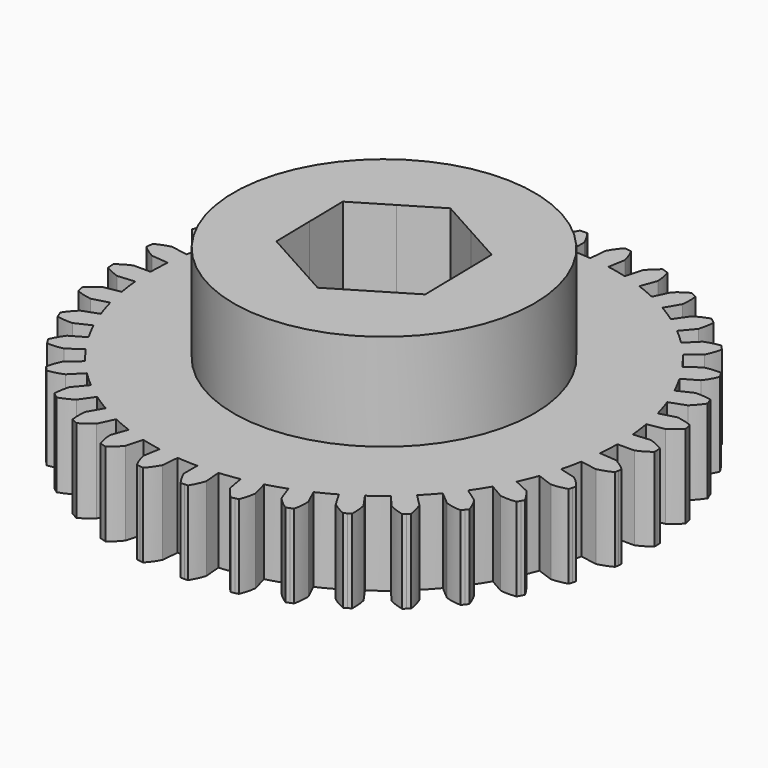
from build123d import *

# Parameters (mm, degrees)
F1_DEPTH = 6.35
F2_R     = 11.43
F3_DEPTH = 7.366
F5_DEPTH = 25.4


with BuildPart() as f1:
    # F0 (on Top) → F1 (new body)
    with BuildSketch(Plane.XY):
        with BuildLine():
            ThreePointArc((0, 19.05), (-0.2695882534, 19.591766176), (-0.6056993608, 20.0949736276))
            ThreePointArc((-0.6056993608, 20.0949736276), (-0.7413308329, 20.0904272082), (-0.8769285255, 20.0849653515))
            ThreePointArc((-0.8769285255, 20.0849653515), (-1.0124862602, 20.0785883065), (-1.1479978601, 20.0712963638))
            ThreePointArc((-1.1479978601, 20.0712963638), (-1.4389725441, 19.5407097553), (-1.6603168993, 18.9775089986))
            Line((-1.6603168993, 18.9775089986), (-1.5474284157, 17.6871877261))
            ThreePointArc((-1.5474284157, 17.6871877261), (-2.3174598996, 17.6028555631), (-3.0830799668, 17.485015364))
            Line((-3.0830799668, 17.485015364), (-3.3079977846, 18.7605876949))
            ThreePointArc((-3.3079977846, 18.7605876949), (-3.6675670958, 19.2473097165), (-4.0859529772, 19.6845072348))
            ThreePointArc((-4.0859529772, 19.6845072348), (-4.218734425, 19.6564777277), (-4.3513236426, 19.6275525567))
            ThreePointArc((-4.3513236426, 19.6275525567), (-4.4837145884, 19.5977330398), (-4.6159012301, 19.5670205357))
            ThreePointArc((-4.6159012301, 19.5670205357), (-4.8103199572, 18.9939675064), (-4.9305028092, 18.4008869908))
            Line((-4.9305028092, 18.4008869908), (-4.5952674177, 17.1497714772))
            ThreePointArc((-4.5952674177, 17.1497714772), (-5.3389562666, 16.9330059453), (-6.0724821089, 16.6840074742))
            Line((-6.0724821089, 16.6840074742), (-6.5154837304, 17.901144426))
            ThreePointArc((-6.5154837304, 17.901144426), (-6.9541087679, 18.3180334907), (-7.44205698, 18.6759370506))
            ThreePointArc((-7.44205698, 18.6759370506), (-7.5679539064, 18.6252761182), (-7.6935059926, 18.5737665096))
            ThreePointArc((-7.6935059926, 18.5737665096), (-7.8187075178, 18.5214105716), (-7.9435527769, 18.46821069))
            ThreePointArc((-7.9435527769, 18.46821069), (-8.0355082324, 17.8701031662), (-8.0508778862, 17.265163343))
            Line((-8.0508778862, 17.265163343), (-7.5034815445, 16.0912681002))
            ThreePointArc((-7.5034815445, 16.0912681002), (-8.1982311492, 15.7486555104), (-8.8773749549, 15.3760644598))
            Line((-8.8773749549, 15.3760644598), (-9.525, 16.4977839421))
            ThreePointArc((-9.525, 16.4977839421), (-10.029353364, 16.8321730868), (-10.5720378473, 17.0999079695))
            ThreePointArc((-10.5720378473, 17.0999079695), (-10.6872249379, 17.0281549187), (-10.8019250562, 16.9556259658))
            ThreePointArc((-10.8019250562, 16.9556259658), (-10.9161329756, 16.8823244155), (-11.0298434923, 16.8082536079))
            ThreePointArc((-11.0298434923, 16.8082536079), (-11.0165416562, 16.203264784), (-10.9266311125, 15.6048464437))
            Line((-10.9266311125, 15.6048464437), (-10.1837061816, 14.5438396845))
            ThreePointArc((-10.1837061816, 14.5438396845), (-10.8084069268, 14.085790147), (-11.4125332551, 13.6009275074))
            Line((-11.4125332551, 13.6009275074), (-12.2451039645, 14.5931466414))
            ThreePointArc((-12.2451039645, 14.5931466414), (-12.7998611333, 14.8348756211), (-13.3807926944, 15.0043068377))
            ThreePointArc((-13.3807926944, 15.0043068377), (-13.4817700477, 14.9136418487), (-13.5821330929, 14.822297307))
            ThreePointArc((-13.5821330929, 14.822297307), (-13.6818772568, 14.7302773748), (-13.7809979945, 14.6375862452))
            ThreePointArc((-13.7809979945, 14.6375862452), (-13.6628430364, 14.0440984006), (-13.4703841816, 13.4703841816))
            Line((-13.4703841816, 13.4703841816), (-12.5545040595, 12.5545040595))
            ThreePointArc((-12.5545040595, 12.5545040595), (-13.0901747293, 11.9949351778), (-13.6009275074, 11.4125332551))
            Line((-13.6009275074, 11.4125332551), (-14.5931466414, 12.2451039645))
            ThreePointArc((-14.5931466414, 12.2451039645), (-15.181451599, 12.3868279664), (-15.7829789264, 12.4528074353))
            ThreePointArc((-15.7829789264, 12.4528074353), (-15.8666783967, 12.3459853177), (-15.9496548885, 12.2386006449))
            ThreePointArc((-15.9496548885, 12.2386006449), (-16.0319046209, 12.1306583101), (-16.1134238461, 12.0221632315))
            ThreePointArc((-16.1134238461, 12.0221632315), (-15.8940058447, 11.4582091939), (-15.6048464437, 10.9266311125))
            Line((-15.6048464437, 10.9266311125), (-14.5438396845, 10.1837061816))
            ThreePointArc((-14.5438396845, 10.1837061816), (-14.9742041965, 9.5396201729), (-15.3760644598, 8.8773749549))
            Line((-15.3760644598, 8.8773749549), (-16.4977839421, 9.525))
            ThreePointArc((-16.4977839421, 9.525), (-17.1017613401, 9.562412812), (-17.7056073303, 9.5229357803))
            ThreePointArc((-17.7056073303, 9.5229357803), (-17.7694857516, 9.4032022702), (-17.8325544913, 9.2830402953))
            ThreePointArc((-17.8325544913, 9.2830402953), (-17.8948106757, 9.1624553309), (-17.956251468, 9.0414528715))
            ThreePointArc((-17.956251468, 9.0414528715), (-17.6422373281, 8.5241680991), (-17.265163343, 8.0508778862))
            Line((-17.265163343, 8.0508778862), (-16.0912681002, 7.5034815445))
            ThreePointArc((-16.0912681002, 7.5034815445), (-16.4032500466, 6.7944486363), (-16.6840074742, 6.0724821089))
            Line((-16.6840074742, 6.0724821089), (-17.901144426, 6.5154837304))
            ThreePointArc((-17.901144426, 6.5154837304), (-18.5024427168, 6.4474485832), (-19.0902598149, 6.3037145405))
            ThreePointArc((-19.0902598149, 6.3037145405), (-19.1323762736, 6.17470768), (-19.1736209495, 6.0454194638))
            ThreePointArc((-19.1736209495, 6.0454194638), (-19.2139919633, 5.915855783), (-19.2534874753, 5.7860225412))
            ThreePointArc((-19.2534874753, 5.7860225412), (-18.8544183577, 5.33112447), (-18.4008869908, 4.9305028092))
            Line((-18.4008869908, 4.9305028092), (-17.1497714772, 4.5952674177))
            ThreePointArc((-17.1497714772, 4.5952674177), (-17.3338914444, 3.8428312161), (-17.485015364, 3.0830799668))
            Line((-17.485015364, 3.0830799668), (-18.7605876949, 3.3079977846))
            ThreePointArc((-18.7605876949, 3.3079977846), (-19.3409367343, 3.1365818917), (-19.8948644153, 2.8929581242))
            ThreePointArc((-19.8948644153, 2.8929581242), (-19.9139392241, 2.7585977215), (-19.9321066375, 2.624111621))
            ThreePointArc((-19.9321066375, 2.624111621), (-19.9493658278, 2.4895059507), (-19.9657160084, 2.3547868439))
            ThreePointArc((-19.9657160084, 2.3547868439), (-19.4937174264, 1.9760973215), (-18.9775089986, 1.6603168993))
            Line((-18.9775089986, 1.6603168993), (-17.6871877261, 1.5474284157))
            ThreePointArc((-17.6871877261, 1.5474284157), (-17.7378513221, 0.7744513139), (-17.7547499098, 0))
            Line((-17.7547499098, 0), (-19.05, 0))
            ThreePointArc((-19.05, 0), (-19.591766176, -0.2695882534), (-20.0949736276, -0.6056993608))
            ThreePointArc((-20.0949736276, -0.6056993608), (-20.0904272082, -0.7413308329), (-20.0849653515, -0.8769285255))
            ThreePointArc((-20.0849653515, -0.8769285255), (-20.0785883065, -1.0124862602), (-20.0712963638, -1.1479978601))
            ThreePointArc((-20.0712963638, -1.1479978601), (-19.5407097553, -1.4389725441), (-18.9775089986, -1.6603168993))
            Line((-18.9775089986, -1.6603168993), (-17.6871877261, -1.5474284157))
            ThreePointArc((-17.6871877261, -1.5474284157), (-17.6028555631, -2.3174598996), (-17.485015364, -3.0830799668))
            Line((-17.485015364, -3.0830799668), (-18.7605876949, -3.3079977846))
            ThreePointArc((-18.7605876949, -3.3079977846), (-19.2473097165, -3.6675670958), (-19.6845072348, -4.0859529772))
            ThreePointArc((-19.6845072348, -4.0859529772), (-19.6564777277, -4.218734425), (-19.6275525567, -4.3513236426))
            ThreePointArc((-19.6275525567, -4.3513236426), (-19.5977330398, -4.4837145884), (-19.5670205357, -4.6159012301))
            ThreePointArc((-19.5670205357, -4.6159012301), (-18.9939675064, -4.8103199572), (-18.4008869908, -4.9305028092))
            Line((-18.4008869908, -4.9305028092), (-17.1497714772, -4.5952674177))
            ThreePointArc((-17.1497714772, -4.5952674177), (-16.9330059453, -5.3389562666), (-16.6840074742, -6.0724821089))
            Line((-16.6840074742, -6.0724821089), (-17.901144426, -6.5154837304))
            ThreePointArc((-17.901144426, -6.5154837304), (-18.3180334907, -6.9541087679), (-18.6759370506, -7.44205698))
            ThreePointArc((-18.6759370506, -7.44205698), (-18.6252761182, -7.5679539064), (-18.5737665096, -7.6935059926))
            ThreePointArc((-18.5737665096, -7.6935059926), (-18.5214105716, -7.8187075178), (-18.46821069, -7.9435527769))
            ThreePointArc((-18.46821069, -7.9435527769), (-17.8701031662, -8.0355082324), (-17.265163343, -8.0508778862))
            Line((-17.265163343, -8.0508778862), (-16.0912681002, -7.5034815445))
            ThreePointArc((-16.0912681002, -7.5034815445), (-15.7486555104, -8.1982311492), (-15.3760644598, -8.8773749549))
            Line((-15.3760644598, -8.8773749549), (-16.4977839421, -9.525))
            ThreePointArc((-16.4977839421, -9.525), (-16.8321730868, -10.029353364), (-17.0999079695, -10.5720378473))
            ThreePointArc((-17.0999079695, -10.5720378473), (-17.0281549187, -10.6872249379), (-16.9556259658, -10.8019250562))
            ThreePointArc((-16.9556259658, -10.8019250562), (-16.8823244155, -10.9161329756), (-16.8082536079, -11.0298434923))
            ThreePointArc((-16.8082536079, -11.0298434923), (-16.203264784, -11.0165416562), (-15.6048464437, -10.9266311125))
            Line((-15.6048464437, -10.9266311125), (-14.5438396845, -10.1837061816))
            ThreePointArc((-14.5438396845, -10.1837061816), (-14.085790147, -10.8084069268), (-13.6009275074, -11.4125332551))
            Line((-13.6009275074, -11.4125332551), (-14.5931466414, -12.2451039645))
            ThreePointArc((-14.5931466414, -12.2451039645), (-14.8348756211, -12.7998611333), (-15.0043068377, -13.3807926944))
            ThreePointArc((-15.0043068377, -13.3807926944), (-14.9136418487, -13.4817700477), (-14.822297307, -13.5821330929))
            ThreePointArc((-14.822297307, -13.5821330929), (-14.7302773748, -13.6818772568), (-14.6375862452, -13.7809979945))
            ThreePointArc((-14.6375862452, -13.7809979945), (-14.0440984006, -13.6628430364), (-13.4703841816, -13.4703841816))
            Line((-13.4703841816, -13.4703841816), (-12.5545040595, -12.5545040595))
            ThreePointArc((-12.5545040595, -12.5545040595), (-11.9949351778, -13.0901747293), (-11.4125332551, -13.6009275074))
            Line((-11.4125332551, -13.6009275074), (-12.2451039645, -14.5931466414))
            ThreePointArc((-12.2451039645, -14.5931466414), (-12.3868279664, -15.181451599), (-12.4528074353, -15.7829789264))
            ThreePointArc((-12.4528074353, -15.7829789264), (-12.3459853177, -15.8666783967), (-12.2386006449, -15.9496548885))
            ThreePointArc((-12.2386006449, -15.9496548885), (-12.1306583101, -16.0319046209), (-12.0221632315, -16.1134238461))
            ThreePointArc((-12.0221632315, -16.1134238461), (-11.4582091939, -15.8940058447), (-10.9266311125, -15.6048464437))
            Line((-10.9266311125, -15.6048464437), (-10.1837061816, -14.5438396845))
            ThreePointArc((-10.1837061816, -14.5438396845), (-9.5396201729, -14.9742041965), (-8.8773749549, -15.3760644598))
            Line((-8.8773749549, -15.3760644598), (-9.525, -16.4977839421))
            ThreePointArc((-9.525, -16.4977839421), (-9.562412812, -17.1017613401), (-9.5229357803, -17.7056073303))
            ThreePointArc((-9.5229357803, -17.7056073303), (-9.4032022702, -17.7694857516), (-9.2830402953, -17.8325544913))
            ThreePointArc((-9.2830402953, -17.8325544913), (-9.1624553309, -17.8948106757), (-9.0414528715, -17.956251468))
            ThreePointArc((-9.0414528715, -17.956251468), (-8.5241680991, -17.6422373281), (-8.0508778862, -17.265163343))
            Line((-8.0508778862, -17.265163343), (-7.5034815445, -16.0912681002))
            ThreePointArc((-7.5034815445, -16.0912681002), (-6.7944486363, -16.4032500466), (-6.0724821089, -16.6840074742))
            Line((-6.0724821089, -16.6840074742), (-6.5154837304, -17.901144426))
            ThreePointArc((-6.5154837304, -17.901144426), (-6.4474485832, -18.5024427168), (-6.3037145405, -19.0902598149))
            ThreePointArc((-6.3037145405, -19.0902598149), (-6.17470768, -19.1323762736), (-6.0454194638, -19.1736209495))
            ThreePointArc((-6.0454194638, -19.1736209495), (-5.915855783, -19.2139919633), (-5.7860225412, -19.2534874753))
            ThreePointArc((-5.7860225412, -19.2534874753), (-5.33112447, -18.8544183577), (-4.9305028092, -18.4008869908))
            Line((-4.9305028092, -18.4008869908), (-4.5952674177, -17.1497714772))
            ThreePointArc((-4.5952674177, -17.1497714772), (-3.8428312161, -17.3338914444), (-3.0830799668, -17.485015364))
            Line((-3.0830799668, -17.485015364), (-3.3079977846, -18.7605876949))
            ThreePointArc((-3.3079977846, -18.7605876949), (-3.1365818917, -19.3409367343), (-2.8929581242, -19.8948644153))
            ThreePointArc((-2.8929581242, -19.8948644153), (-2.7585977215, -19.9139392241), (-2.624111621, -19.9321066375))
            ThreePointArc((-2.624111621, -19.9321066375), (-2.4895059507, -19.9493658278), (-2.3547868439, -19.9657160084))
            ThreePointArc((-2.3547868439, -19.9657160084), (-1.9760973215, -19.4937174264), (-1.6603168993, -18.9775089986))
            Line((-1.6603168993, -18.9775089986), (-1.5474284157, -17.6871877261))
            ThreePointArc((-1.5474284157, -17.6871877261), (-0.7744513139, -17.7378513221), (0, -17.7547499098))
            Line((0, -17.7547499098), (0, -19.05))
            ThreePointArc((0, -19.05), (0.2695882534, -19.591766176), (0.6056993608, -20.0949736276))
            ThreePointArc((0.6056993608, -20.0949736276), (0.7413308329, -20.0904272082), (0.8769285255, -20.0849653515))
            ThreePointArc((0.8769285255, -20.0849653515), (1.0124862602, -20.0785883065), (1.1479978601, -20.0712963638))
            ThreePointArc((1.1479978601, -20.0712963638), (1.4389725441, -19.5407097553), (1.6603168993, -18.9775089986))
            Line((1.6603168993, -18.9775089986), (1.5474284157, -17.6871877261))
            ThreePointArc((1.5474284157, -17.6871877261), (2.3174598996, -17.6028555631), (3.0830799668, -17.485015364))
            Line((3.0830799668, -17.485015364), (3.3079977846, -18.7605876949))
            ThreePointArc((3.3079977846, -18.7605876949), (3.6675670958, -19.2473097165), (4.0859529772, -19.6845072348))
            ThreePointArc((4.0859529772, -19.6845072348), (4.218734425, -19.6564777277), (4.3513236426, -19.6275525567))
            ThreePointArc((4.3513236426, -19.6275525567), (4.4837145884, -19.5977330398), (4.6159012301, -19.5670205357))
            ThreePointArc((4.6159012301, -19.5670205357), (4.8103199572, -18.9939675064), (4.9305028092, -18.4008869908))
            Line((4.9305028092, -18.4008869908), (4.5952674177, -17.1497714772))
            ThreePointArc((4.5952674177, -17.1497714772), (5.3389562666, -16.9330059453), (6.0724821089, -16.6840074742))
            Line((6.0724821089, -16.6840074742), (6.5154837304, -17.901144426))
            ThreePointArc((6.5154837304, -17.901144426), (6.9541087679, -18.3180334907), (7.44205698, -18.6759370506))
            ThreePointArc((7.44205698, -18.6759370506), (7.5679539064, -18.6252761182), (7.6935059926, -18.5737665096))
            ThreePointArc((7.6935059926, -18.5737665096), (7.8187075178, -18.5214105716), (7.9435527769, -18.46821069))
            ThreePointArc((7.9435527769, -18.46821069), (8.0355082324, -17.8701031662), (8.0508778862, -17.265163343))
            Line((8.0508778862, -17.265163343), (7.5034815445, -16.0912681002))
            ThreePointArc((7.5034815445, -16.0912681002), (8.1982311492, -15.7486555104), (8.8773749549, -15.3760644598))
            Line((8.8773749549, -15.3760644598), (9.525, -16.4977839421))
            ThreePointArc((9.525, -16.4977839421), (10.029353364, -16.8321730868), (10.5720378473, -17.0999079695))
            ThreePointArc((10.5720378473, -17.0999079695), (10.6872249379, -17.0281549187), (10.8019250562, -16.9556259658))
            ThreePointArc((10.8019250562, -16.9556259658), (10.9161329756, -16.8823244155), (11.0298434923, -16.8082536079))
            ThreePointArc((11.0298434923, -16.8082536079), (11.0165416562, -16.203264784), (10.9266311125, -15.6048464437))
            Line((10.9266311125, -15.6048464437), (10.1837061816, -14.5438396845))
            ThreePointArc((10.1837061816, -14.5438396845), (10.8084069268, -14.085790147), (11.4125332551, -13.6009275074))
            Line((11.4125332551, -13.6009275074), (12.2451039645, -14.5931466414))
            ThreePointArc((12.2451039645, -14.5931466414), (12.7998611333, -14.8348756211), (13.3807926944, -15.0043068377))
            ThreePointArc((13.3807926944, -15.0043068377), (13.4817700477, -14.9136418487), (13.5821330929, -14.822297307))
            ThreePointArc((13.5821330929, -14.822297307), (13.6818772568, -14.7302773748), (13.7809979945, -14.6375862452))
            ThreePointArc((13.7809979945, -14.6375862452), (13.6628430364, -14.0440984006), (13.4703841816, -13.4703841816))
            Line((13.4703841816, -13.4703841816), (12.5545040595, -12.5545040595))
            ThreePointArc((12.5545040595, -12.5545040595), (13.0901747293, -11.9949351778), (13.6009275074, -11.4125332551))
            Line((13.6009275074, -11.4125332551), (14.5931466414, -12.2451039645))
            ThreePointArc((14.5931466414, -12.2451039645), (15.181451599, -12.3868279664), (15.7829789264, -12.4528074353))
            ThreePointArc((15.7829789264, -12.4528074353), (15.8666783967, -12.3459853177), (15.9496548885, -12.2386006449))
            ThreePointArc((15.9496548885, -12.2386006449), (16.0319046209, -12.1306583101), (16.1134238461, -12.0221632315))
            ThreePointArc((16.1134238461, -12.0221632315), (15.8940058447, -11.4582091939), (15.6048464437, -10.9266311125))
            Line((15.6048464437, -10.9266311125), (14.5438396845, -10.1837061816))
            ThreePointArc((14.5438396845, -10.1837061816), (14.9742041965, -9.5396201729), (15.3760644598, -8.8773749549))
            Line((15.3760644598, -8.8773749549), (16.4977839421, -9.525))
            ThreePointArc((16.4977839421, -9.525), (17.1017613401, -9.562412812), (17.7056073303, -9.5229357803))
            ThreePointArc((17.7056073303, -9.5229357803), (17.7694857516, -9.4032022702), (17.8325544913, -9.2830402953))
            ThreePointArc((17.8325544913, -9.2830402953), (17.8948106757, -9.1624553309), (17.956251468, -9.0414528715))
            ThreePointArc((17.956251468, -9.0414528715), (17.6422373281, -8.5241680991), (17.265163343, -8.0508778862))
            Line((17.265163343, -8.0508778862), (16.0912681002, -7.5034815445))
            ThreePointArc((16.0912681002, -7.5034815445), (16.4032500466, -6.7944486363), (16.6840074742, -6.0724821089))
            Line((16.6840074742, -6.0724821089), (17.901144426, -6.5154837304))
            ThreePointArc((17.901144426, -6.5154837304), (18.5024427168, -6.4474485832), (19.0902598149, -6.3037145405))
            ThreePointArc((19.0902598149, -6.3037145405), (19.1323762736, -6.17470768), (19.1736209495, -6.0454194638))
            ThreePointArc((19.1736209495, -6.0454194638), (19.2139919633, -5.915855783), (19.2534874753, -5.7860225412))
            ThreePointArc((19.2534874753, -5.7860225412), (18.8544183577, -5.33112447), (18.4008869908, -4.9305028092))
            Line((18.4008869908, -4.9305028092), (17.1497714772, -4.5952674177))
            ThreePointArc((17.1497714772, -4.5952674177), (17.3338914444, -3.8428312161), (17.485015364, -3.0830799668))
            Line((17.485015364, -3.0830799668), (18.7605876949, -3.3079977846))
            ThreePointArc((18.7605876949, -3.3079977846), (19.3409367343, -3.1365818917), (19.8948644153, -2.8929581242))
            ThreePointArc((19.8948644153, -2.8929581242), (19.9139392241, -2.7585977215), (19.9321066375, -2.624111621))
            ThreePointArc((19.9321066375, -2.624111621), (19.9493658278, -2.4895059507), (19.9657160084, -2.3547868439))
            ThreePointArc((19.9657160084, -2.3547868439), (19.4937174264, -1.9760973215), (18.9775089986, -1.6603168993))
            Line((18.9775089986, -1.6603168993), (17.6871877261, -1.5474284157))
            ThreePointArc((17.6871877261, -1.5474284157), (17.7378513221, -0.7744513139), (17.7547499098, 0))
            Line((17.7547499098, 0), (19.05, 0))
            ThreePointArc((19.05, 0), (19.591766176, 0.2695882534), (20.0949736276, 0.6056993608))
            ThreePointArc((20.0949736276, 0.6056993608), (20.0904272082, 0.7413308329), (20.0849653515, 0.8769285255))
            ThreePointArc((20.0849653515, 0.8769285255), (20.0785883065, 1.0124862602), (20.0712963638, 1.1479978601))
            ThreePointArc((20.0712963638, 1.1479978601), (19.5407097553, 1.4389725441), (18.9775089986, 1.6603168993))
            Line((18.9775089986, 1.6603168993), (17.6871877261, 1.5474284157))
            ThreePointArc((17.6871877261, 1.5474284157), (17.6028555631, 2.3174598996), (17.485015364, 3.0830799668))
            Line((17.485015364, 3.0830799668), (18.7605876949, 3.3079977846))
            ThreePointArc((18.7605876949, 3.3079977846), (19.2473097165, 3.6675670958), (19.6845072348, 4.0859529772))
            ThreePointArc((19.6845072348, 4.0859529772), (19.6564777277, 4.218734425), (19.6275525567, 4.3513236426))
            ThreePointArc((19.6275525567, 4.3513236426), (19.5977330398, 4.4837145884), (19.5670205357, 4.6159012301))
            ThreePointArc((19.5670205357, 4.6159012301), (18.9939675064, 4.8103199572), (18.4008869908, 4.9305028092))
            Line((18.4008869908, 4.9305028092), (17.1497714772, 4.5952674177))
            ThreePointArc((17.1497714772, 4.5952674177), (16.9330059453, 5.3389562666), (16.6840074742, 6.0724821089))
            Line((16.6840074742, 6.0724821089), (17.901144426, 6.5154837304))
            ThreePointArc((17.901144426, 6.5154837304), (18.3180334907, 6.9541087679), (18.6759370506, 7.44205698))
            ThreePointArc((18.6759370506, 7.44205698), (18.6252761182, 7.5679539064), (18.5737665096, 7.6935059926))
            ThreePointArc((18.5737665096, 7.6935059926), (18.5214105716, 7.8187075178), (18.46821069, 7.9435527769))
            ThreePointArc((18.46821069, 7.9435527769), (17.8701031662, 8.0355082324), (17.265163343, 8.0508778862))
            Line((17.265163343, 8.0508778862), (16.0912681002, 7.5034815445))
            ThreePointArc((16.0912681002, 7.5034815445), (15.7486555104, 8.1982311492), (15.3760644598, 8.8773749549))
            Line((15.3760644598, 8.8773749549), (16.4977839421, 9.525))
            ThreePointArc((16.4977839421, 9.525), (16.8321730868, 10.029353364), (17.0999079695, 10.5720378473))
            ThreePointArc((17.0999079695, 10.5720378473), (17.0281549187, 10.6872249379), (16.9556259658, 10.8019250562))
            ThreePointArc((16.9556259658, 10.8019250562), (16.8823244155, 10.9161329756), (16.8082536079, 11.0298434923))
            ThreePointArc((16.8082536079, 11.0298434923), (16.203264784, 11.0165416562), (15.6048464437, 10.9266311125))
            Line((15.6048464437, 10.9266311125), (14.5438396845, 10.1837061816))
            ThreePointArc((14.5438396845, 10.1837061816), (14.085790147, 10.8084069268), (13.6009275074, 11.4125332551))
            Line((13.6009275074, 11.4125332551), (14.5931466414, 12.2451039645))
            ThreePointArc((14.5931466414, 12.2451039645), (14.8348756211, 12.7998611333), (15.0043068377, 13.3807926944))
            ThreePointArc((15.0043068377, 13.3807926944), (14.9136418487, 13.4817700477), (14.822297307, 13.5821330929))
            ThreePointArc((14.822297307, 13.5821330929), (14.7302773748, 13.6818772568), (14.6375862452, 13.7809979945))
            ThreePointArc((14.6375862452, 13.7809979945), (14.0440984006, 13.6628430364), (13.4703841816, 13.4703841816))
            Line((13.4703841816, 13.4703841816), (12.5545040595, 12.5545040595))
            ThreePointArc((12.5545040595, 12.5545040595), (11.9949351778, 13.0901747293), (11.4125332551, 13.6009275074))
            Line((11.4125332551, 13.6009275074), (12.2451039645, 14.5931466414))
            ThreePointArc((12.2451039645, 14.5931466414), (12.3868279664, 15.181451599), (12.4528074353, 15.7829789264))
            ThreePointArc((12.4528074353, 15.7829789264), (12.3459853177, 15.8666783967), (12.2386006449, 15.9496548885))
            ThreePointArc((12.2386006449, 15.9496548885), (12.1306583101, 16.0319046209), (12.0221632315, 16.1134238461))
            ThreePointArc((12.0221632315, 16.1134238461), (11.4582091939, 15.8940058447), (10.9266311125, 15.6048464437))
            Line((10.9266311125, 15.6048464437), (10.1837061816, 14.5438396845))
            ThreePointArc((10.1837061816, 14.5438396845), (9.5396201729, 14.9742041965), (8.8773749549, 15.3760644598))
            Line((8.8773749549, 15.3760644598), (9.525, 16.4977839421))
            ThreePointArc((9.525, 16.4977839421), (9.562412812, 17.1017613401), (9.5229357803, 17.7056073303))
            ThreePointArc((9.5229357803, 17.7056073303), (9.4032022702, 17.7694857516), (9.2830402953, 17.8325544913))
            ThreePointArc((9.2830402953, 17.8325544913), (9.1624553309, 17.8948106757), (9.0414528715, 17.956251468))
            ThreePointArc((9.0414528715, 17.956251468), (8.5241680991, 17.6422373281), (8.0508778862, 17.265163343))
            Line((8.0508778862, 17.265163343), (7.5034815445, 16.0912681002))
            ThreePointArc((7.5034815445, 16.0912681002), (6.7944486363, 16.4032500466), (6.0724821089, 16.6840074742))
            Line((6.0724821089, 16.6840074742), (6.5154837304, 17.901144426))
            ThreePointArc((6.5154837304, 17.901144426), (6.4474485832, 18.5024427168), (6.3037145405, 19.0902598149))
            ThreePointArc((6.3037145405, 19.0902598149), (6.17470768, 19.1323762736), (6.0454194638, 19.1736209495))
            ThreePointArc((6.0454194638, 19.1736209495), (5.915855783, 19.2139919633), (5.7860225412, 19.2534874753))
            ThreePointArc((5.7860225412, 19.2534874753), (5.33112447, 18.8544183577), (4.9305028092, 18.4008869908))
            Line((4.9305028092, 18.4008869908), (4.5952674177, 17.1497714772))
            ThreePointArc((4.5952674177, 17.1497714772), (3.8428312161, 17.3338914444), (3.0830799668, 17.485015364))
            Line((3.0830799668, 17.485015364), (3.3079977846, 18.7605876949))
            ThreePointArc((3.3079977846, 18.7605876949), (3.1365818917, 19.3409367343), (2.8929581242, 19.8948644153))
            ThreePointArc((2.8929581242, 19.8948644153), (2.7585977215, 19.9139392241), (2.624111621, 19.9321066375))
            ThreePointArc((2.624111621, 19.9321066375), (2.4895059507, 19.9493658278), (2.3547868439, 19.9657160084))
            ThreePointArc((2.3547868439, 19.9657160084), (1.9760973215, 19.4937174264), (1.6603168993, 18.9775089986))
            Line((1.6603168993, 18.9775089986), (1.5474284157, 17.6871877261))
            ThreePointArc((1.5474284157, 17.6871877261), (0.7744513139, 17.7378513221), (0, 17.7547499098))
            Line((0, 17.7547499098), (0, 19.05))
        make_face()
    extrude(amount=-F1_DEPTH)

    # F2 (on face) → F3 (join)
    with BuildSketch(Plane.XY):
        Circle(F2_R)
    extrude(amount=F3_DEPTH)

    # F4 (on face) → F5 (cut)
    with BuildSketch(Plane.XY.offset(7.366)):
        with BuildLine():
            ThreePointArc((2.8755042101, -4.7913692759), (4.8628212761, -2.752946283), (5.588, 0))
            ThreePointArc((5.588, 0), (5.5877999003, 0.0472892602), (5.5871996156, 0.0945751337))
            ThreePointArc((5.5871996156, 0.0945751337), (4.791369266, 2.8755042265), (2.7116954406, 4.8859443138))
            ThreePointArc((2.7116954406, 4.8859443138), (-0.0945750171, 5.5871996175), (-2.8755041753, 4.7913692967))
            ThreePointArc((-2.8755041753, 4.7913692967), (-4.8859443157, 2.7116954372), (-5.5871996174, -0.0945750277))
            ThreePointArc((-5.5871996174, -0.0945750277), (-4.7913692667, -2.8755042255), (-2.7116953501, -4.885944364))
            ThreePointArc((-2.7116953501, -4.885944364), (0.0945750891, -5.5871996163), (2.8755042101, -4.7913692759))
        make_face()
        with BuildLine():
            ThreePointArc((5.5871996156, 0.0945751337), (5.5877999003, 0.0472892602), (5.588, 0))
            ThreePointArc((5.588, 0), (4.8628212761, -2.752946283), (2.8755042101, -4.7913692759))
            Line((2.8755042101, -4.7913692759), (5.6418025499, -3.1311961486))
            Line((5.6418025499, -3.1311961486), (5.5871996156, 0.0945751337))
        make_face()
        with BuildLine():
            ThreePointArc((2.7116954406, 4.8859443138), (4.791369266, 2.8755042265), (5.5871996156, 0.0945751337))
            Line((5.5871996156, 0.0945751337), (5.5325966839, 3.320346257))
            Line((5.5325966839, 3.320346257), (2.7116954406, 4.8859443138))
        make_face()
        with BuildLine():
            Line((0.109205866, -6.4515424057), (2.8755042101, -4.7913692759))
            ThreePointArc((2.8755042101, -4.7913692759), (0.0945750891, -5.5871996163), (-2.7116953501, -4.885944364))
            Line((-2.7116953501, -4.885944364), (0.109205866, -6.4515424057))
        make_face()
        with BuildLine():
            ThreePointArc((-2.8755041753, 4.7913692967), (-0.0945750171, 5.5871996175), (2.7116954406, 4.8859443138))
            Line((2.7116954406, 4.8859443138), (-0.109205866, 6.4515424057))
            Line((-0.109205866, 6.4515424057), (-2.8755041753, 4.7913692967))
        make_face()
        with BuildLine():
            Line((-5.5325966839, -3.320346257), (-2.7116953501, -4.885944364))
            ThreePointArc((-2.7116953501, -4.885944364), (-4.7913692667, -2.8755042255), (-5.5871996174, -0.0945750277))
            Line((-5.5871996174, -0.0945750277), (-5.5325966839, -3.320346257))
        make_face()
        with BuildLine():
            ThreePointArc((-5.5871996174, -0.0945750277), (-4.8859443157, 2.7116954372), (-2.8755041753, 4.7913692967))
            Line((-2.8755041753, 4.7913692967), (-5.6418025499, 3.1311961486))
            Line((-5.6418025499, 3.1311961486), (-5.5871996174, -0.0945750277))
        make_face()
    extrude(amount=-F5_DEPTH, mode=Mode.SUBTRACT)


solid = f1.part
